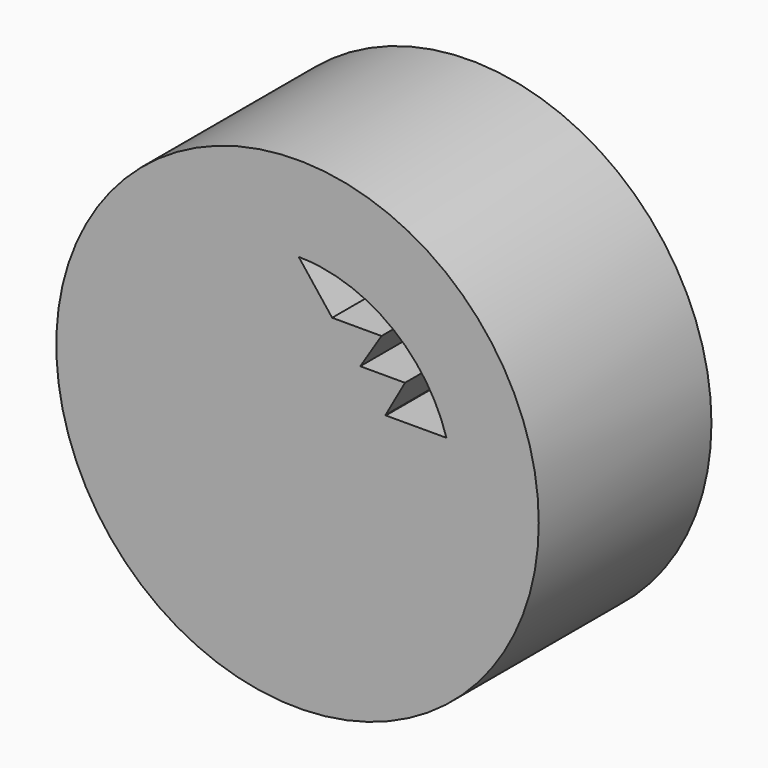
from build123d import *

# Parameters (mm, degrees)
F0_R     = 52.0995656
F1_DEPTH = 25.4
F2_R     = 3665.7043167314
F3_DEPTH = 3280


# Not quite as in the source:
# - the dataset's text gives a spline's control points without its knots; the knots are read off the source's solid


with BuildPart() as f1:
    # F0 (on Front) → F1 (new body)
    with BuildSketch(Plane.XZ):
        with BuildLine():
            Line((-526.8820044, 1723.750045), (-19.7821804, 2372.922229))
            add(Edge.make_bspline(
                [(-19.7821804, 2372.922229), (-79.064739, 2372.423119), (-211.5361276, 2366.2951658), (-417.926774, 2339.1526242), (-638.4698432, 2288.5473406), (-858.5238862, 2214.9105308), (-1074.602753, 2117.773641), (-1283.0525012, 1997.3756344), (-1480.2288404, 1854.7141468), (-1662.6955062, 1691.5456136), (-1827.4117884, 1510.317909), (-1971.9018728, 1314.0537854), (-2094.3753896, 1106.1833604), (-2192.0399898, 894.1563016), (-2242.35137, 749.8136134), (-2263.2966164, 679.3982348)],
                knots=[587.035817, 587.035817, 587.035817, 587.035817, 594.037943, 602.687578, 611.595752, 620.732399, 630.061528, 639.54174, 649.127101, 658.768332, 668.414253, 678.013386, 687.515595, 696.873625, 705.550536, 705.550536, 705.550536, 705.550536], degree=3))
            Line((-2263.2966164, 679.3982348), (-1342.206993, 679.998386))
            Line((-1342.206993, 679.998386), (-1339.882258, 682.9744278))
            Line((-1339.882258, 682.9744278), (-1638.4439926, 1213.9828908))
            Line((-1638.4439926, 1213.9828908), (-965.6990592, 1213.9116438))
            Line((-965.6990592, 1213.9116438), (-1291.9168472, 1723.9302326))
            Line((-1291.9168472, 1723.9302326), (-526.8820044, 1723.750045))
        make_face()
        with BuildLine():
            Line((1840.7334026, 44.2460634), (2299.7240772, -542.0645242))
            add(Edge.make_bspline(
                [(2299.7240772, -542.0645242), (2307.1285328, -510.3627334), (2329.1476404, -406.527889), (2354.2915322, -230.8312122), (2365.3225236, -14.9792436), (2357.0012296, 200.9952546), (2329.0220882, 415.6879164), (2297.1922814, 557.4054892), (2278.389398, 626.4230804)],
                knots=[418.30978, 418.30978, 418.30978, 418.30978, 422.154862, 430.84382, 439.25032, 447.656865, 456.345961, 464.794751, 464.794751, 464.794751, 464.794751], degree=3))
            Line((2278.389398, 626.4230804), (1840.7334026, 44.2460634))
        make_face()
        with BuildLine():
            Line((-1839.7216698, 43.096815), (-2278.1857408, 627.1695102))
            add(Edge.make_bspline(
                [(-2278.1857408, 627.1695102), (-2294.4544662, 567.529218), (-2324.9974582, 435.5281612), (-2354.291583, 230.8311868), (-2365.3223966, 14.979269), (-2357.001382, -200.99528), (-2332.6479382, -387.8660264), (-2309.0012748, -502.5715628), (-2299.0540506, -544.9250468)],
                knots=[707.688753, 707.688753, 707.688753, 707.688753, 714.990257, 723.679215, 732.085715, 740.49226, 749.181356, 754.319852, 754.319852, 754.319852, 754.319852], degree=3))
            Line((-2299.0540506, -544.9250468), (-1839.7216698, 43.096815))
        make_face()
        Polygon((-1387.7701226, -558.9423416), (-1816.0289562, 11.536045), (-2261.6891774, -558.9832102), align=None)
        Polygon((1817.030402, 12.7159512), (1387.3794452, -558.8125984), (2264.4169088, -558.7716028), align=None)
        Polygon((974.079078, 38.3814066), (1318.843565, -558.8157988), (1339.7125606, -558.8148336), (1792.714982, 43.7762396), (1323.1181564, 643.6350348), (1313.2235864, 643.6286086), align=None)
        Polygon((-1322.9415756, -558.939319), (-976.9536722, 37.4859804), (-1316.7964012, 641.9149468), (-1323.612923, 641.9105018), (-1791.7349738, 42.6363638), (-1340.1307716, -558.9401318), align=None)
        Polygon((-559.7679178, -1661.9141006), (-896.6562712, -1213.1491866), (-1118.5026906, -1661.8939584), align=None)
        Polygon((481.779072, -1700.0516672), (-483.5231122, -1700.0168438), (-1.1982958, -2342.515889), align=None)
        with BuildLine():
            Line((1358.7364748, -596.9139446), (1348.6124412, -610.3811008))
            Line((1348.6124412, -610.3811008), (1683.577659, -1190.6041466))
            Line((1683.577659, -1190.6041466), (923.1375492, -1190.607093))
            Line((923.1375492, -1190.607093), (1174.1587134, -1700.07661))
            Line((1174.1587134, -1700.07661), (529.4430102, -1700.053369))
            Line((529.4430102, -1700.053369), (23.6355382, -2372.886542))
            add(Edge.make_bspline(
                [(23.6355382, -2372.886542), (81.6327552, -2372.3032056), (212.8110806, -2366.1276528), (417.9266724, -2339.152421), (638.4698432, -2288.5474676), (858.5239116, -2214.9105562), (1074.6026768, -2117.773514), (1283.0524504, -1997.3756344), (1480.229069, -1854.7143754), (1662.6952014, -1691.5454104), (1827.4118392, -1510.3180106), (1971.9019998, -1314.0538108), (2094.3751864, -1106.183335), (2193.791777, -890.3534136), (2253.0674014, -718.8408534), (2280.132981, -620.4658914), (2286.2368296, -596.8705614)],
                knots=[294.352137, 294.352137, 294.352137, 294.352137, 301.202548, 309.852184, 318.760357, 327.897005, 337.226133, 346.706345, 356.291707, 365.932938, 375.578859, 385.177992, 394.6802, 404.038231, 413.209047, 416.087635, 416.087635, 416.087635, 416.087635], degree=3))
            Line((2286.2368296, -596.8705614), (1358.7364748, -596.9139446))
        make_face()
        Polygon((-478.5445344, 1723.7386658), (477.7401164, 1723.513444), (-1.0091166, 2335.0634528), align=None)
        Polygon((-922.5742026, 1217.1982006), (-556.6383076, 1685.6570554), (-1222.309849, 1685.8138496), align=None)
        with BuildLine():
            Line((-1351.2015902, -607.654868), (-1359.1694178, -597.0410208))
            Line((-1359.1694178, -597.0410208), (-2286.1816354, -597.0843532))
            add(Edge.make_bspline(
                [(-2286.1816354, -597.0843532), (-2282.5917772, -610.9562076), (-2258.7446316, -699.7927076), (-2204.7911454, -862.4982496), (-2108.091161, -1079.5703326), (-1988.2360032, -1288.9752986), (-1846.2204376, -1487.0541252), (-1683.7912984, -1670.3534538), (-1503.3869602, -1835.8201282), (-1308.016307, -1980.967463), (-1101.0940132, -2103.9959952), (-886.251085, -2203.8616324), (-667.1385438, -2280.2796914), (-447.2478482, -2333.673895), (-233.452162, -2364.5491952), (-93.1738548, -2372.1169982), (-26.0591808, -2372.8610404)],
                knots=[170.764235, 170.764235, 170.764235, 170.764235, 172.456617, 181.627765, 190.986213, 200.488911, 210.088586, 219.735076, 229.376877, 238.962781, 248.443484, 257.773032, 266.910011, 275.818422, 284.468196, 292.395615, 292.395615, 292.395615, 292.395615], degree=3))
            Line((-26.0591808, -2372.8610404), (-531.165435, -1700.015142))
            Line((-531.165435, -1700.015142), (-1179.8387376, -1699.9917486))
            Line((-1179.8387376, -1699.9917486), (-928.0172956, -1190.6142812))
            Line((-928.0172956, -1190.6142812), (-1689.3796032, -1190.617253))
            Line((-1689.3796032, -1190.617253), (-1351.2015902, -607.654868))
        make_face()
        Polygon((23.1786684, 1685.520505), (295.51757, 1213.7780906), (876.832384, 1213.716521), (507.5720354, 1685.4064082), align=None)
        with BuildLine():
            Line((17.7265838, 2372.9387644), (526.1352444, 1723.5020394))
            Line((526.1352444, 1723.5020394), (1275.7075578, 1723.3255094))
            Line((1275.7075578, 1723.3255094), (952.9407916, 1213.7084692))
            Line((952.9407916, 1213.7084692), (1632.622084, 1213.636511))
            Line((1632.622084, 1213.636511), (1337.5388286, 687.0223242))
            Line((1337.5388286, 687.0223242), (1341.6684876, 681.7471506))
            Line((1341.6684876, 681.7471506), (2262.4171922, 682.3470732))
            add(Edge.make_bspline(
                [(2262.4171922, 682.3470732), (2244.5283532, 742.2030368), (2198.6072614, 876.3790956), (2108.0911864, 1079.5702818), (1988.2361556, 1288.9755018), (1846.220209, 1487.0538712), (1683.7913746, 1670.3534792), (1503.3869856, 1835.8202806), (1308.0162054, 1980.9672344), (1101.0940386, 2103.9960714), (886.251085, 2203.8616324), (667.1385184, 2280.2796406), (447.2478482, 2333.6739204), (230.6999958, 2364.9465528), (87.6210592, 2372.4117652), (17.7265838, 2372.9387644)],
                knots=[467.084579, 467.084579, 467.084579, 467.084579, 474.463159, 483.821608, 493.324306, 502.923981, 512.570471, 522.212272, 531.798176, 541.278879, 550.608426, 559.745406, 568.653816, 577.303591, 585.559079, 585.559079, 585.559079, 585.559079], degree=3))
        make_face()
        Polygon((615.7226192, 681.2741264), (1290.890738, 681.7140544), (1291.8992196, 683.5138476), (918.9064172, 1159.9715434), align=None)
        Polygon((1371.4797056, 643.6665562), (1816.4179826, 75.3063518), (2244.1145618, 644.2351352), align=None)
        Polygon((1567.6033164, 1175.5433944), (955.0515062, 1175.6082406), (1312.084625, 719.537296), align=None)
        Polygon((285.425642, -1190.6095822), (21.3228936, -1661.9350556), (510.4202644, -1661.9526832), (864.757732, -1190.6073216), align=None)
        Polygon((-316.6478554, 1175.7429114), (-896.0978522, 1175.8042778), (-592.2169512, 700.7078442), align=None)
        Polygon((1.1006582, 1647.5592398), (-250.5033852, 1213.835901), (251.5216712, 1213.7827388), align=None)
        Polygon((317.5141986, 1175.6757538), (587.5269936, 707.9625922), (883.7159364, 1175.6158098), align=None)
        Polygon((-1573.3088676, 1175.875982), (-1314.4665862, 715.5107356), (-954.9041354, 1175.8105008), align=None)
        Polygon((-21.7384122, 1175.7116948), (-272.6039252, 1175.7382378), (-559.8882376, 680.5081386), (-286.712533, 680.6861164), align=None)
        Polygon((951.9166128, 76.7709666), (1269.5339608, 643.6001352), (624.9262076, 643.1801208), align=None)
        Polygon((1206.4884176, 1685.2417908), (555.9671634, 1685.3950036), (915.6159742, 1225.9828414), align=None)
        Polygon((-954.757552, 75.7484134), (-626.0617654, 642.3650094), (-1273.1030418, 641.9434202), align=None)
        Polygon((639.427474, -558.8475742), (1274.851527, -558.8178562), (952.410465, -0.2890266), align=None)
        Polygon((-641.6289682, -558.9074674), (-955.2744674, -1.0716768), (-1278.8937592, -558.9372616), align=None)
        Polygon((-20.9185002, 1685.5308936), (-508.3008122, 1685.6456762), (-876.8024628, 1213.9022204), (-294.54729, 1213.8405746), align=None)
        Polygon((-624.4968968, 680.4660254), (-925.6751616, 1151.3370674), (-1293.835995, 680.0299074), align=None)
        Polygon((630.6352386, -596.9479806), (900.023854, -1143.6957822), (1303.0242164, -607.6182666), (1296.8462252, -596.9168402), align=None)
        Polygon((1323.7285438, -643.4820506), (941.0651486, -1152.5070168), (1617.5892972, -1152.5044006), align=None)
        Polygon((-1300.9962804, -597.038303), (-1305.5881432, -604.9539336), (-903.3656558, -1140.7496616), (-634.5550936, -597.0071372), align=None)
        Polygon((861.8917484, -1152.5073216), (602.1592986, -625.3574742), (306.7746722, -1152.5094806), align=None)
        Polygon((893.2380408, -1216.1273874), (558.0841772, -1661.9544104), (1112.9117188, -1661.9744256), align=None)
        Polygon((241.7518914, -1190.6097346), (-242.741323, -1190.6116396), (-0.0822706, -1622.1940632), align=None)
        Polygon((-605.225993, -623.6521436), (-866.680004, -1152.5140526), (-307.8724094, -1152.5118936), align=None)
        Polygon((-286.4505574, -1190.611792), (-865.9324058, -1190.6140526), (-512.125595, -1661.9158278), (-21.4479632, -1661.9335062), align=None)
        Polygon((-942.1749254, -1152.5143574), (-1326.3550562, -640.7526174), (-1623.2309166, -1152.516999), align=None)
        Polygon((-1815.4276874, 74.1971592), (-1371.983921, 641.8789804), (-2241.1619642, 641.3126366), align=None)
        Polygon((-607.39147, -542.0612984), (-479.6169224, -283.6025062), (-752.7007806, -283.6206926), align=None)
        Polygon((-933.0783472, 37.1907562), (-778.4074348, -237.8999814), (-619.9332026, 58.1621138), (-756.7617834, 341.131017), align=None)
        Polygon((774.0501156, -240.6548146), (930.2480252, 38.1005334), (754.2905158, 342.8921514), (615.3394602, 57.0498732), align=None)
        Polygon((-554.9293702, 642.4113644), (-420.0639046, 431.5586492), (-307.1135844, 642.5728322), align=None)
        Polygon((282.672282, 681.0571342), (558.9625092, 681.237144), (273.5182998, 1175.6804274), (18.9671706, 1175.7073768), align=None)
        Polygon((-243.482622, 680.714285), (239.511205, 681.028991), (-1.4135608, 1132.9485342), align=None)
        Polygon((-263.883648, 642.6010008), (-389.4787232, 407.9638272), (-137.7785916, 407.8585696), (-21.650706, 642.7588364), align=None)
        Polygon((263.1009216, -1152.5096584), (574.4031438, -596.9506222), (297.4164232, -596.9635508), (27.358975, -1152.5105728), align=None)
        Polygon((-576.4994566, -597.0044194), (-264.1631496, -1152.5117158), (-34.5167458, -1152.5108268), (-303.1359952, -596.9916432), align=None)
        Polygon((-3.570097, -1128.9891568), (255.0523728, -596.965532), (-260.8164964, -596.989662), align=None)
        Polygon((441.8126292, -299.9198218), (315.9376714, -558.8626872), (569.3907586, -558.8508508), align=None)
        Polygon((414.21304, 434.316886), (546.4645408, 643.1289906), (302.9768896, 642.9703422), align=None)
        Polygon((-445.9919198, -301.5578932), (-573.216532, -558.904267), (-321.5587168, -558.8925068), align=None)
        Polygon((-739.2712672, -245.5197782), (-473.0975044, -245.5020744), (-599.4228296, 15.7455362), align=None)
        Polygon((-450.2154572, 407.9892272), (-590.6290702, 627.5160678), (-717.912204, 408.1011904), align=None)
        Polygon((-728.4035216, 370.0055846), (-597.6986522, 99.7008166), (-453.073262, 369.890421), align=None)
        Polygon((-254.2341626, 172.2954898), (-156.6102278, 369.7664436), (-380.600331, 369.8601188), align=None)
        Polygon((-412.3558936, -283.5980358), (-279.2391926, -558.8905256), (-39.518717, -558.8793242), (-254.8248904, -283.5875456), align=None)
        Polygon((-0.9388348, 598.6831308), (-95.2857378, 407.840815), (93.1300906, 407.7620242), align=None)
        Polygon((385.2588688, 407.6398502), (259.8158126, 642.9422244), (19.8049134, 642.7858366), (135.6124796, 407.7442442), align=None)
        Polygon((733.415348, -245.4217596), (594.7469944, 14.6882104), (468.2961424, -245.4394126), align=None)
        Polygon((476.2151766, -283.5388792), (604.325563, -543.5501702), (750.030631, -283.5206674), align=None)
        Polygon((251.4899212, -283.5538398), (37.646356, -558.8757174), (273.573621, -558.8646684), (407.4102596, -283.5434766), align=None)
        Polygon((724.8121394, 369.3978388), (448.7607484, 369.5132818), (593.1811098, 98.6138998), align=None)
        Polygon((250.1507824, 175.2786944), (373.1896016, 369.5449048), (154.3886168, 369.6363956), align=None)
        Polygon((-392.5516406, -107.4892694), (-554.5291424, 99.616133), (-577.1882792, 57.284239), (-445.6130534, -214.8204238), align=None)
        Polygon((-525.1037758, 154.5886926), (-288.0964774, 154.5276056), (-417.1425998, 356.2821424), align=None)
        Polygon((28.7685226, -245.4686734), (232.8390568, -245.4550844), (344.2820902, -101.9730498), (245.9946312, 97.5099904), align=None)
        Polygon((-32.2485004, -245.4727374), (-249.9784434, 94.9327286), (-347.7777144, -102.8929108), (-236.255179, -245.486301), align=None)
        Polygon((-284.6214018, -245.4895268), (-366.5106716, -140.7854182), (-418.2777512, -245.4984168), align=None)
        Polygon((586.0175224, 634.372747), (442.4007408, 407.6159488), (716.9914794, 407.5011154), align=None)
        Polygon((111.9062532, 369.6541502), (-114.1173994, 369.748689), (-220.5250606, 154.5102066), (217.9657058, 154.397202), align=None)
        Polygon((281.0838676, -245.451884), (414.9712808, -245.4429686), (363.006894, -139.9766568), align=None)
        Polygon((203.2451104, -283.5570656), (-206.4586676, -283.5843198), (-0.90805, -546.4025902), align=None)
        Polygon((-373.8186834, -69.5967874), (-281.854402, 116.4260054), (-519.3552986, 116.4872194), align=None)
        Polygon((572.588644, 56.252237), (549.3196278, 99.8995208), (388.994777, -106.51744), (441.5818702, -213.2475288), align=None)
        Polygon((-1.7493234, -222.4467992), (212.7955866, 116.2985228), (-218.4884886, 116.4096732), align=None)
        with Locations((-0.774827, 2.0098512)):
            Circle(F0_R, mode=Mode.SUBTRACT)
        Polygon((279.2193806, 116.2814032), (370.2699986, -68.513833), (513.754243, 116.2209512), align=None)
        Polygon((520.307697, 154.3192748), (411.3815496, 358.6396942), (282.0137616, 154.380692), align=None)
    extrude(amount=F1_DEPTH)


with BuildPart() as f3:
    # F2 (on face) → F3 (new body)
    with BuildSketch(Plane.XZ.offset(25.4)):
        Circle(F2_R)
        with BuildLine():
            Line((1632.622084, 1213.636511), (952.9407916, 1213.7084692))
            Line((952.9407916, 1213.7084692), (1275.7075578, 1723.3255094))
            Line((1275.7075578, 1723.3255094), (526.1352444, 1723.5020394))
            Line((526.1352444, 1723.5020394), (17.7265838, 2372.9387644))
            add(Edge.make_bspline(
                [(2262.4171922, 682.3470732), (2244.5283532, 742.2030368), (2198.6072614, 876.3790956), (2108.0911864, 1079.5702818), (1988.2361556, 1288.9755018), (1846.220209, 1487.0538712), (1683.7913746, 1670.3534792), (1503.3869856, 1835.8202806), (1308.0162054, 1980.9672344), (1101.0940386, 2103.9960714), (886.251085, 2203.8616324), (667.1385184, 2280.2796406), (447.2478482, 2333.6739204), (230.6999958, 2364.9465528), (87.6210592, 2372.4117652), (17.7265838, 2372.9387644)],
                knots=[467.084579, 467.084579, 467.084579, 467.084579, 474.463159, 483.821608, 493.324306, 502.923981, 512.570471, 522.212272, 531.798176, 541.278879, 550.608426, 559.745406, 568.653816, 577.303591, 585.559079, 585.559079, 585.559079, 585.559079], degree=3))
            Line((2262.4171922, 682.3470732), (1341.6684876, 681.7471506))
            Line((1341.6684876, 681.7471506), (1337.5388286, 687.0223242))
            Line((1337.5388286, 687.0223242), (1632.622084, 1213.636511))
        make_face(mode=Mode.SUBTRACT)
    extrude(amount=F3_DEPTH)


solid = Compound([f1.part, f3.part])
